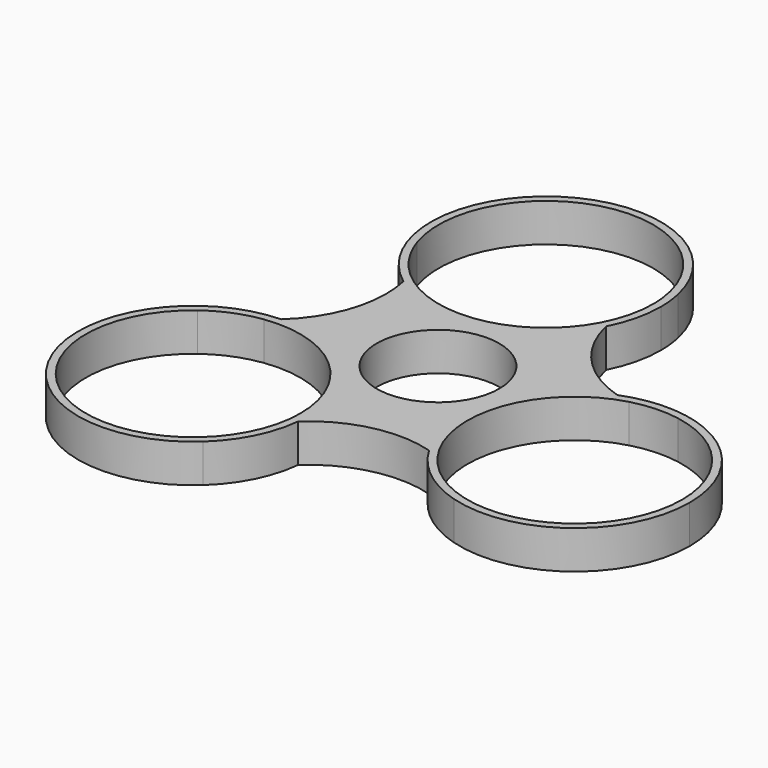
from build123d import *

# Parameters (mm, degrees)
F0_R     = 8
F1_DEPTH = 5


# Not quite as in the source:
# - a feature names something its author has since deleted; it is built from what else it names


with BuildPart() as f1:
    # F0 (on Top) → F1 (new body)
    with BuildSketch(Plane.XY):
        with BuildLine():
            ThreePointArc((7.9121440123, 17.5499293192), (9.1490120469, 20.8777196251), (9.5691464087, 24.4029881218))
            ThreePointArc((9.5691464087, 24.4029881218), (9.4793257017, 26.042059033), (9.2109392818, 27.6615002765))
            ThreePointArc((9.2109392818, 27.6615002765), (8.8193827537, 26.8385345747), (8.4785274274, 25.9933087425))
            ThreePointArc((8.4785274274, 25.9933087425), (8.5464733038, 25.1994382891), (8.5691464087, 24.4029881218))
            ThreePointArc((8.5691464087, 24.4029881218), (8.3311107472, 21.8323194251), (7.6250981876, 19.3490665605))
            ThreePointArc((7.6250981876, 19.3490665605), (7.7412805882, 18.4451358603), (7.9121440123, 17.5499293192))
        make_face()
        with BuildLine():
            ThreePointArc((8.4785274274, 25.9933087425), (8.8193827537, 26.8385345747), (9.2109392818, 27.6615002765))
            ThreePointArc((9.2109392818, 27.6615002765), (-8.689365746, 39.0447809948), (-20.0726464643, 21.144475967))
            ThreePointArc((-20.0726464643, 21.144475967), (-19.3800207125, 20.593183388), (-18.7211221359, 20.0019925512))
            ThreePointArc((-18.7211221359, 20.0019925512), (-8.442463209, 38.0752303486), (8.4785274274, 25.9933087425))
        make_face()
        with BuildLine():
            ThreePointArc((18.2808163885, 6.4299700246), (11.5832094425, 10.578918544), (7.9121440123, 17.5499293192))
            ThreePointArc((7.9121440123, 17.5499293192), (-2.0581580843, 9.7870747046), (-14.4218573571, 12.3962462122))
            ThreePointArc((-14.4218573571, 12.3962462122), (-14.7542295678, 4.6387919255), (-18.9207994891, -1.9131744502))
            ThreePointArc((-18.9207994891, -1.9131744502), (-7.9907957387, -6.1219111722), (-3.4181808461, -16.9047512351))
            ThreePointArc((-3.4181808461, -16.9047512351), (-3.4376551817, -17.6688525497), (-3.4960276219, -18.4309698155))
            ThreePointArc((-3.4960276219, -18.4309698155), (3.2731601147, -14.8661881946), (10.919943616, -15.1034068738))
            ThreePointArc((10.919943616, -15.1034068738), (9.655402449, -2.646349524), (18.2808163885, 6.4299700246))
        make_face()
        Circle(F0_R, mode=Mode.SUBTRACT)
        with BuildLine():
            ThreePointArc((-14.4218573571, 12.3962462122), (-2.0581580843, 9.7870747046), (7.9121440123, 17.5499293192))
            ThreePointArc((7.9121440123, 17.5499293192), (7.7412805882, 18.4451358603), (7.6250981876, 19.3490665605))
            ThreePointArc((7.6250981876, 19.3490665605), (-2.2534030631, 10.7683334455), (-14.907533277, 14.0980115505))
            ThreePointArc((-14.907533277, 14.0980115505), (-14.6395764677, 13.2542976843), (-14.4218573571, 12.3962462122))
        make_face()
        with BuildLine():
            ThreePointArc((-18.7211221359, 20.0019925512), (-19.3800207125, 20.593183388), (-20.0726464643, 21.144475967))
            ThreePointArc((-20.0726464643, 21.144475967), (-18.0308595518, 16.2642013697), (-14.4218573571, 12.3962462122))
            ThreePointArc((-14.4218573571, 12.3962462122), (-14.6395764677, 13.2542976843), (-14.907533277, 14.0980115505))
            ThreePointArc((-14.907533277, 14.0980115505), (-17.1908591544, 16.8067871532), (-18.7211221359, 20.0019925512))
        make_face()
        with BuildLine():
            ThreePointArc((20.1455918313, 6.0030413071), (19.2063911412, 6.1867474035), (18.2808163885, 6.4299700246))
            ThreePointArc((18.2808163885, 6.4299700246), (9.655402449, -2.646349524), (10.919943616, -15.1034068738))
            ThreePointArc((10.919943616, -15.1034068738), (11.7048264649, -15.3603839917), (12.474376183, -15.6601698438))
            ThreePointArc((12.474376183, -15.6601698438), (10.6520286886, -2.8250110982), (20.1455918313, 6.0030413071))
        make_face()
        with BuildLine():
            ThreePointArc((28.1221549341, 6.8802345627), (23.1634660922, 7.4860881247), (18.2808163885, 6.4299700246))
            ThreePointArc((18.2808163885, 6.4299700246), (19.2063911412, 6.1867474035), (20.1455918313, 6.0030413071))
            ThreePointArc((20.1455918313, 6.0030413071), (23.2091706485, 6.4871331239), (26.3041545683, 6.2848101329))
            ThreePointArc((26.3041545683, 6.2848101329), (27.2226565904, 6.5535105265), (28.1221549341, 6.8802345627))
        make_face()
        with BuildLine():
            ThreePointArc((-20.2929169032, -3.0308417387), (-19.5903609061, -2.4922611868), (-18.9207994891, -1.9131744502))
            ThreePointArc((-18.9207994891, -1.9131744502), (-24.0938941246, -3.0200013713), (-28.5610315871, -5.8538427275))
            ThreePointArc((-28.5610315871, -5.8538427275), (-27.6775469435, -5.7980858959), (-26.7988899679, -5.6903090014))
            ThreePointArc((-26.7988899679, -5.6903090014), (-23.7155132394, -3.9456513623), (-20.2929169032, -3.0308417387))
        make_face()
        with BuildLine():
            ThreePointArc((-3.4181808461, -16.9047512351), (-7.9907957387, -6.1219111722), (-18.9207994891, -1.9131744502))
            ThreePointArc((-18.9207994891, -1.9131744502), (-19.5903609061, -2.4922611868), (-20.2929169032, -3.0308417387))
            ThreePointArc((-20.2929169032, -3.0308417387), (-9.2053176863, -6.3632545482), (-4.4181808461, -16.9047512351))
            ThreePointArc((-4.4181808461, -16.9047512351), (-4.4869248616, -18.2904303809), (-4.6924818025, -19.6625013626))
            ThreePointArc((-4.6924818025, -19.6625013626), (-4.1118905803, -19.0296020384), (-3.4960276219, -18.4309698155))
            ThreePointArc((-3.4960276219, -18.4309698155), (-3.4376551817, -17.6688525497), (-3.4181808461, -16.9047512351))
        make_face()
        with BuildLine():
            ThreePointArc((38.8490344373, -7.4982368866), (35.8718628785, 1.471244496), (28.1221549341, 6.8802345627))
            ThreePointArc((28.1221549341, 6.8802345627), (27.2226565904, 6.5535105265), (26.3041545683, 6.2848101329))
            ThreePointArc((26.3041545683, 6.2848101329), (34.5815011117, 1.4914326892), (37.8490344373, -7.4982368866))
            ThreePointArc((37.8490344373, -7.4982368866), (31.7032518121, -19.0875107823), (18.6617102331, -20.5017620856))
            ThreePointArc((18.6617102331, -20.5017620856), (19.1377449469, -21.1766467253), (19.5759139405, -21.876708336))
            ThreePointArc((19.5759139405, -21.876708336), (32.81851582, -19.5210653278), (38.8490344373, -7.4982368866))
        make_face()
        with BuildLine():
            ThreePointArc((12.474376183, -15.6601698438), (11.7048264649, -15.3603839917), (10.919943616, -15.1034068738))
            ThreePointArc((10.919943616, -15.1034068738), (14.6052028869, -19.311431978), (19.5759139405, -21.876708336))
            ThreePointArc((19.5759139405, -21.876708336), (19.1377449469, -21.1766467253), (18.6617102331, -20.5017620856))
            ThreePointArc((18.6617102331, -20.5017620856), (15.2214583236, -18.5238856386), (12.474376183, -15.6601698438))
        make_face()
        with BuildLine():
            ThreePointArc((-26.7988899679, -5.6903090014), (-27.6775469435, -5.7980858959), (-28.5610315871, -5.8538427275))
            ThreePointArc((-28.5610315871, -5.8538427275), (-29.4690893537, -27.0476019762), (-8.275330105, -27.9556597428))
            ThreePointArc((-8.275330105, -27.9556597428), (-8.1635176407, -27.1041048739), (-8.003150447, -26.2603453792))
            ThreePointArc((-8.003150447, -26.2603453792), (-28.7533738733, -26.348467934), (-26.7988899679, -5.6903090014))
        make_face()
        with BuildLine():
            ThreePointArc((-8.275330105, -27.9556597428), (-5.0113342557, -23.6320437442), (-3.4960276219, -18.4309698155))
            ThreePointArc((-3.4960276219, -18.4309698155), (-4.1118905803, -19.0296020384), (-4.6924818025, -19.6625013626))
            ThreePointArc((-4.6924818025, -19.6625013626), (-5.9051240284, -23.183557577), (-8.003150447, -26.2603453792))
            ThreePointArc((-8.003150447, -26.2603453792), (-8.1635176407, -27.1041048739), (-8.275330105, -27.9556597428))
        make_face()
    extrude(amount=F1_DEPTH)


solid = f1.part
